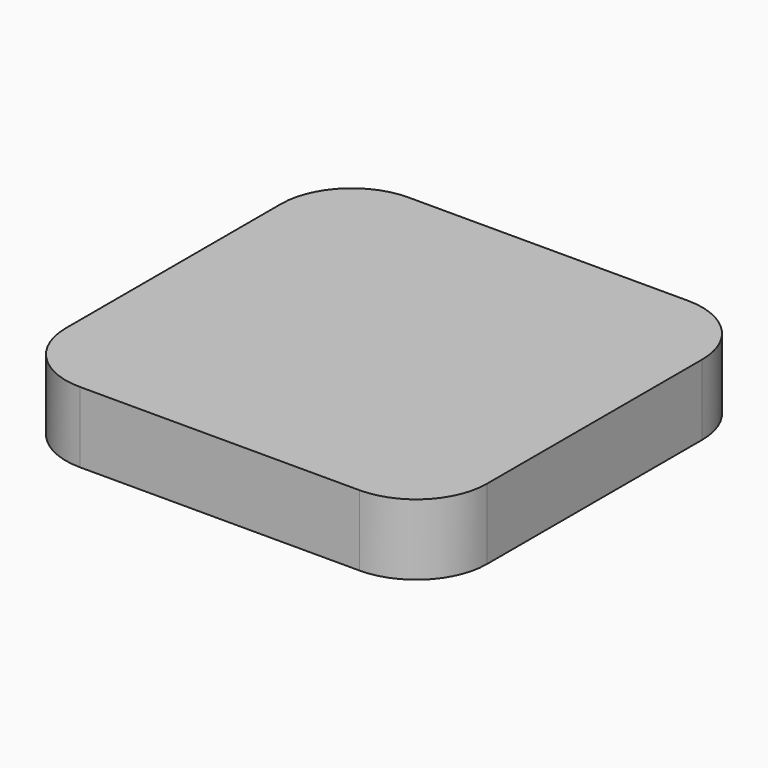
from build123d import *

# Parameters (mm, degrees)
F0_W     = 29.766542837
F0_H     = 29.0134996176
F1_DEPTH = 5
F4_R     = 5


# Not quite as in the source:
# - the program builds the solid bodies; features that only make, move or delete a surface that nothing else refers to are left out


with BuildPart() as f1:
    # F0 (on Top) → F1 (new body)
    with BuildSketch(Plane.XY):
        Rectangle(F0_W, F0_H)
    extrude(amount=F1_DEPTH)

    # F4
    f4_edges = [f1.edges().sort_by_distance(p)[0] for p in [
        (14.883271, 14.50675, 2.5),
        (14.883271, -14.50675, 2.5),
        (-14.883271, 14.50675, 2.5),
        (-14.883271, -14.50675, 2.5),
    ]]
    fillet(f4_edges, radius=F4_R)


solid = f1.part
